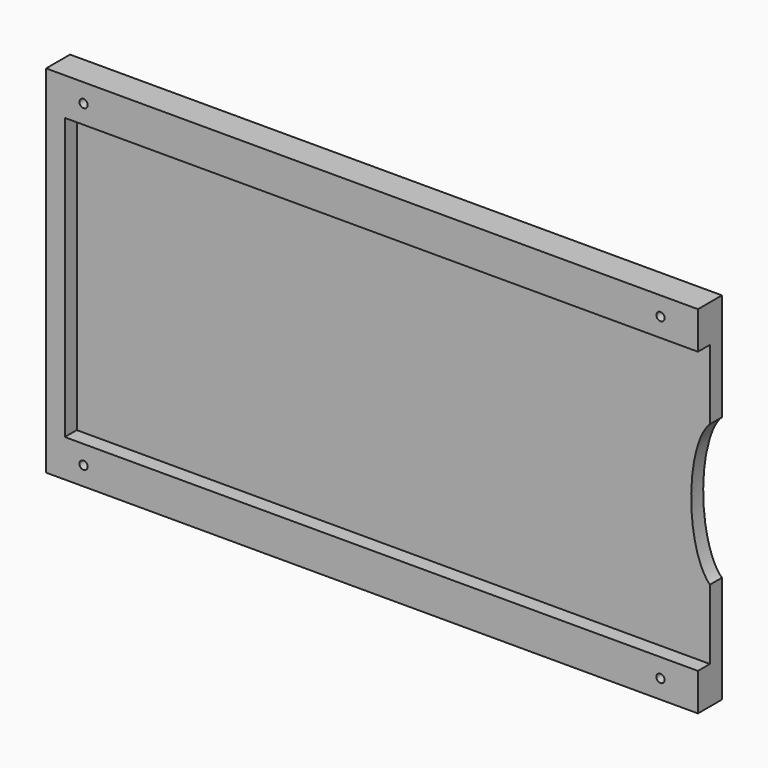
from build123d import *

# Parameters (mm, degrees)
F0_W     = 220.98
F0_H     = 120.65
F0_R     = 1.397
F1_DEPTH = 5.08
F2_W     = 214.63
F2_H     = 12.7
F2_R     = 1.397
F2_W_2   = 6.35
F2_H_2   = 95.25
F3_DEPTH = 5.08
F5_DEPTH = 25.4


# Not quite as in the source:
# - a feature names something its author has since deleted; it is built from what else it names


with BuildPart() as f1:
    # F0 (on Front) → F1 (new body)
    with BuildSketch(Plane.XZ):
        with Locations((110.49, 60.325)):
            Rectangle(F0_W, F0_H)
        with Locations((12.7, 6.35)):
            Circle(F0_R, mode=Mode.SUBTRACT)
        with Locations((208.28, 6.35)):
            Circle(F0_R, mode=Mode.SUBTRACT)
        with Locations((12.7, 114.3)):
            Circle(F0_R, mode=Mode.SUBTRACT)
        with Locations((208.28, 114.3)):
            Circle(F0_R, mode=Mode.SUBTRACT)
    extrude(amount=F1_DEPTH)

    # F2 (on face) → F3 (join)
    with BuildSketch(Plane.XZ.offset(5.08)):
        with Locations((113.665, 114.3)):
            Rectangle(F2_W, F2_H)
        with Locations((12.7, 114.3)):
            Circle(F2_R, mode=Mode.SUBTRACT)
        with Locations((208.28, 114.3)):
            Circle(F2_R, mode=Mode.SUBTRACT)
        with Locations((113.665, 6.35)):
            Rectangle(F2_W, F2_H)
        with Locations((12.7, 6.35)):
            Circle(F2_R, mode=Mode.SUBTRACT)
        with Locations((208.28, 6.35)):
            Circle(F2_R, mode=Mode.SUBTRACT)
        with Locations((3.175, 60.325)):
            Rectangle(F2_W_2, F2_H_2)
        with Locations((3.175, 114.3)):
            Rectangle(F2_W_2, F2_H)
        with Locations((3.175, 6.35)):
            Rectangle(F2_W_2, F2_H)
    extrude(amount=F3_DEPTH)

    # F4 (on face) → F5 (cut)
    with BuildSketch(Plane.XZ.offset(5.08)):
        with BuildLine():
            add(Edge.make_bspline(
                [(224.155, 85.725), (207.6572160579, 85.725), (215.906108029, 47.625), (224.155, 9.525), (232.403891971, 47.625), (240.6527839421, 85.725), (224.155, 85.725)],
                knots=[0, 0, 0, 2.0943951024, 2.0943951024, 4.1887902048, 4.1887902048, 6.2831853072, 6.2831853072, 6.2831853072], degree=2, weights=[1, 0.5, 1, 0.5, 1, 0.5, 1]))
        make_face()
    extrude(amount=-F5_DEPTH, mode=Mode.SUBTRACT)


solid = f1.part
